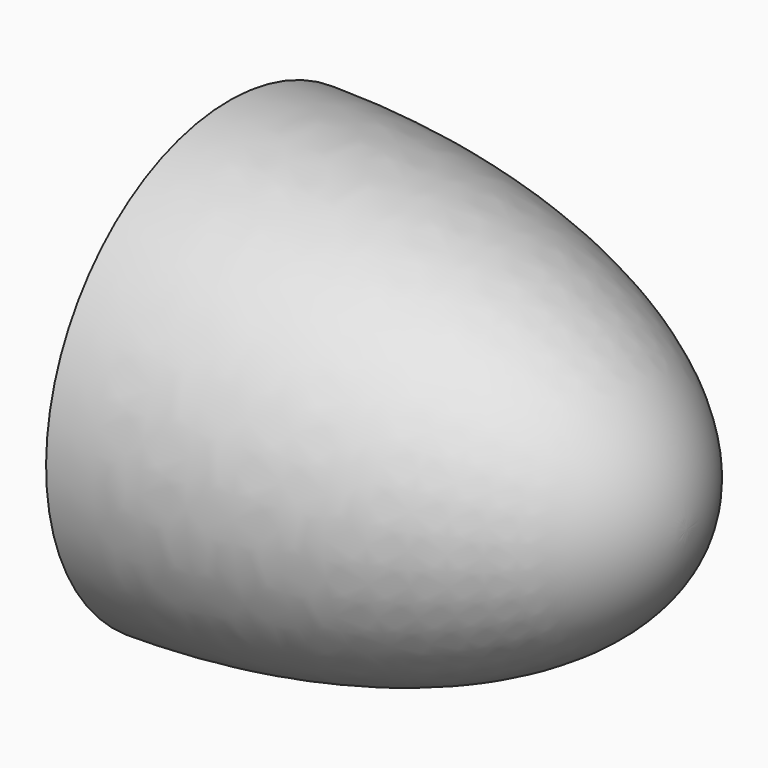
from build123d import *

# Parameters (mm, degrees)
F1_R     = 50.8
F3_DEPTH = 125


# Not quite as in the source:
# - an extrude ends at something that could not be found from the text; its depth is read off the source's solid


with BuildPart() as f2:
    # F0 (on Top) → F2 (revolve)
    with BuildSketch(Plane.XY):
        with BuildLine():
            add(Edge.make_bspline(
                [(50.8, 0), (50.8, 25.4), (0, 25.4), (-50.8, 25.4), (-50.8, 0)],
                knots=[3.1415926536, 3.1415926536, 3.1415926536, 4.7123889804, 4.7123889804, 6.2831853072, 6.2831853072, 6.2831853072], degree=2, weights=[1, 0.7071067812, 1, 0.7071067812, 1]))
            Line((-50.8, 0), (50.8, 0))
        make_face()
    revolve(axis=Axis((0, 0, 0), (1, 0, 0)))

    # F1 (on Right) → F3 (cut, through all)
    with BuildSketch(Plane.YZ):
        Circle(F1_R)
    extrude(amount=-F3_DEPTH, mode=Mode.SUBTRACT)


solid = f2.part
